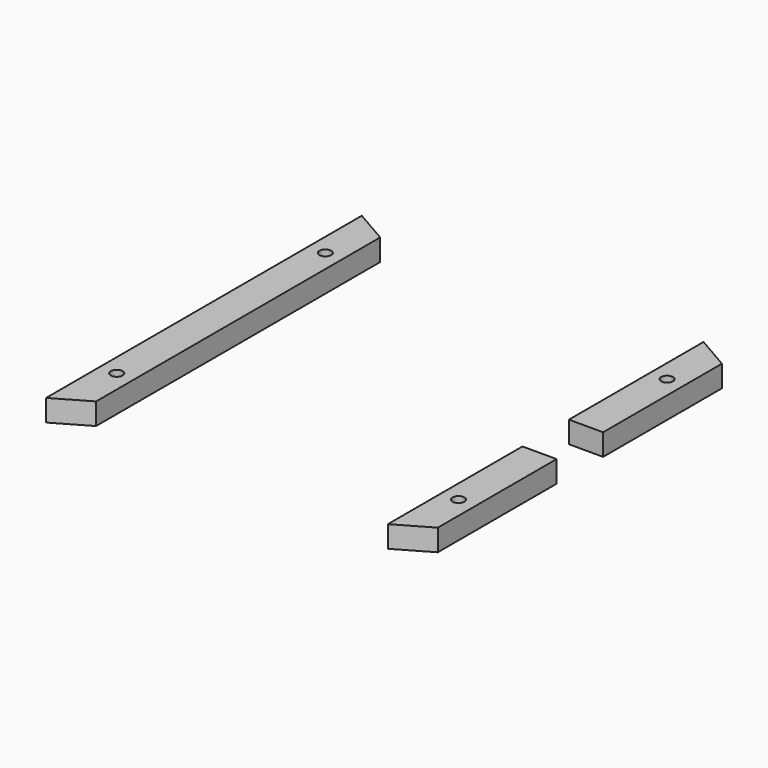
from build123d import *

# Parameters (mm, degrees)
F0_R     = 1.7272
F1_DEPTH = 6.35


# Not quite as in the source:
# - a length typed as a fraction of an inch, garbled in the dataset ("3 / 203.2 mm" for 3/8 in), is restored


with BuildPart() as f1:
    # F0 (on Top) → F1 (new body)
    with BuildSketch(Plane.XY):
        Polygon((0, 115.47), (0, 0), (10, 5.7735026919), (10, 109.6964973081), align=None)
        with Locations((5, 19.5867513459)):
            Circle(F0_R, mode=Mode.SUBTRACT)
        with Locations((5, 95.8832486541)):
            Circle(F0_R, mode=Mode.SUBTRACT)
    extrude(amount=F1_DEPTH)


with BuildPart() as f1b:
    # F0 (on Top) → F1, piece 2 (new body)
    with BuildSketch(Plane.XY):
        Polygon((100, 49.235), (100, 0), (110, 5.7735026919), (110, 49.235), align=None)
        with Locations((105, 19.5867513459)):
            Circle(F0_R, mode=Mode.SUBTRACT)
    extrude(amount=F1_DEPTH)


with BuildPart() as f1c:
    # F0 (on Top) → F1, piece 3 (new body)
    with BuildSketch(Plane.XY):
        Polygon((110, 109.6964973081), (100, 115.47), (100, 66.235), (110, 66.235), align=None)
        with Locations((105, 95.8832486541)):
            Circle(F0_R, mode=Mode.SUBTRACT)
    extrude(amount=F1_DEPTH)


solid = Compound([f1.part, f1b.part, f1c.part])
